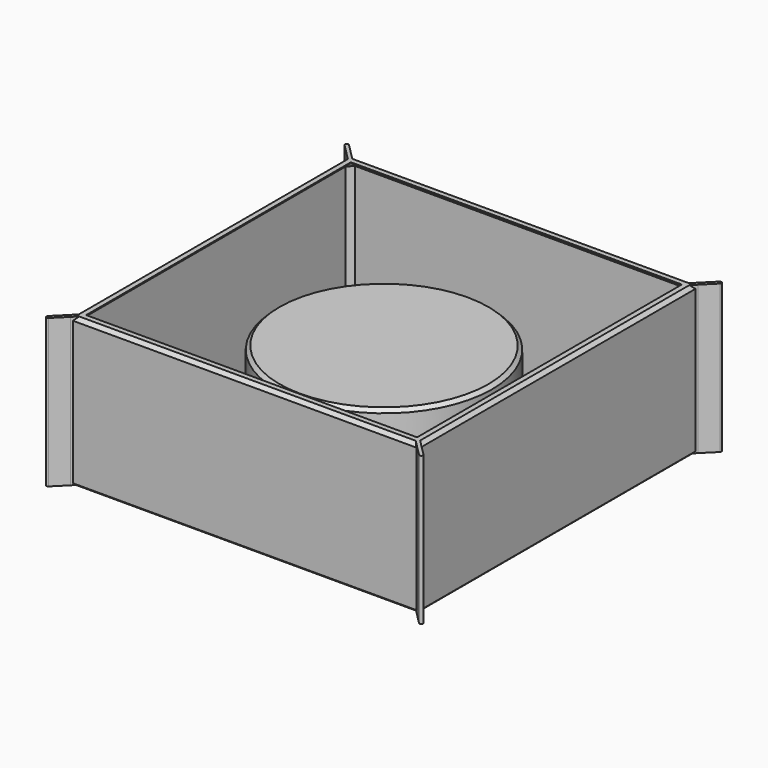
from build123d import *

# Parameters (mm, degrees)
F0_W             = 80
F0_H             = 80
F1_DEPTH         = 34
F2_T             = -0.8
F3_R             = 25
F4_DEPTH         = 24
F4_TAPER         = 0.5
F5_T1_DEPTH      = 78.4
F5_T3_DEPTH      = 78.4
F6_W             = 80
F6_H             = 80
F6_W_2           = 76
F6_H_2           = 76
F7_DEPTH         = 0.05
F8_SIZE          = 1.19999
F11_DEPTH        = 34.05
F11_COPIES_COUNT = 4
F14_SIZE         = 3
F16_SIZE         = 0.4
F17_SIZE         = 0.8


# Not quite as in the source:
# - a fillet or chamfer that OpenCascade refuses, or shapes differently, is made with other operations: its cross-section is extruded or revolved along the edge and cut away or added
# - a fillet or chamfer is up to 0.001 mm smaller than in the source, because OpenCascade refuses the exact size
# - a pattern or mirror of a feature is missing from the dataset's text; its kind, count and spacing are read off the source's solid


with BuildPart() as f1:
    # F0 (on Top) → F1 (new body)
    with BuildSketch(Plane.XY):
        Rectangle(F0_W, F0_H)
    extrude(amount=F1_DEPTH)

    # F2
    f2_openings = [f1.faces().sort_by_distance(p)[0] for p in [
        (0, 0, 34),
    ]]
    offset(amount=F2_T, openings=f2_openings)

    # F3 (on face) → F4 (join)
    with BuildSketch(Plane.XY.offset(0.8)):
        Circle(F3_R)
    extrude(amount=F4_DEPTH, taper=F4_TAPER)

    # F5: chamfer of 1.2 on 5 edges, made by hand

    # F5_s2 → F5_t1 (join)
    with BuildSketch(Plane.XZ.offset(-39.2)):
        Polygon((-39.2, 2), (-38, 0.8), (-39.2, 0.8), align=None)
        Polygon((39.2, 2), (38, 0.8), (39.2, 0.8), align=None)
    extrude(amount=F5_T1_DEPTH)

    # F5_s4 → F5_t3 (join)
    with BuildSketch(Plane.YZ.offset(-39.2)):
        Polygon((-39.2, 2), (-38, 0.8), (-39.2, 0.8), align=None)
        Polygon((39.2, 2), (38, 0.8), (39.2, 0.8), align=None)
    extrude(amount=F5_T3_DEPTH)

    # F5_s5 → F5_t6 (revolve)
    with BuildSketch(Plane.XZ):
        Polygon((26.1895734527, 0.8), (24.989619145, 1.9895281574), (25, 0.8), align=None)
    revolve(axis=Axis((0, 0, 0.8), (0, 0, -1)))

    # F6 (on face) → F7 (join)
    with BuildSketch(Plane.XY.offset(34)):
        Rectangle(F6_W, F6_H)
        Rectangle(F6_W_2, F6_H_2, mode=Mode.SUBTRACT)
    extrude(amount=F7_DEPTH)

    # F8 (size 1.2 in the source; OpenCascade refuses exactly that, so slightly less here)
    f8_edges = [f1.edges().sort_by_distance(p)[0] for p in [
        (0, -39.2, 34),
        (-39.2, 0, 34),
        (-39.2, -39.2, 18),
        (-39.2, 39.2, 18),
        (0, 39.2, 34),
        (39.2, 0, 34),
        (39.2, 39.2, 18),
        (39.2, -39.2, 18),
    ]]
    chamfer(f8_edges, length=F8_SIZE)

    # F9: chamfer of 0.8 on 1 edges, made by hand

    # F9_s1 → F9_t2 (revolve, cut)
    with BuildSketch(Plane.XZ):
        Polygon((24.7975364014, 24.0000304615), (23.990555173, 24.8), (24.790555173, 24.8), align=None)
    revolve(axis=Axis((0, 0, 24.8), (0, 0, -1)), mode=Mode.SUBTRACT)

    # F10 (on face) → F11 (join, through all)
    with BuildSketch(Plane(origin=(0, 0, 0), x_dir=(1, 0, 0), z_dir=(0, 0, -1))):
        with BuildLine():
            Line((-39.1612012219, 39.7268866468), (-39.7171572875, 40.2828427125))
            ThreePointArc((-39.7171572875, 40.2828427125), (-39.7171572875, 39.7171572875), (-40.2828427125, 39.7171572875))
            Line((-40.2828427125, 39.7171572875), (-39.7268866468, 39.1612012219))
            Line((-39.7268866468, 39.1612012219), (-39.1612012219, 39.7268866468))
        make_face()
        with BuildLine():
            ThreePointArc((-40.2828427125, 39.7171572875), (-39.7171572875, 39.7171572875), (-39.7171572875, 40.2828427125))
            Line((-39.7171572875, 40.2828427125), (-42.5455844123, 43.1112698372))
            ThreePointArc((-42.5455844123, 43.1112698372), (-43.1112698372, 43.1112698372), (-43.1112698372, 42.5455844123))
            Line((-43.1112698372, 42.5455844123), (-40.2828427125, 39.7171572875))
        make_face()
    f11 = extrude(amount=-F11_DEPTH)

    # F11_copies: F11 ×4 about axis
    f11_copies_axis = Axis((0, 0, 0), (0, 0, 1))
    for i in range(1, F11_COPIES_COUNT):
        add(f11.rotate(f11_copies_axis, i * 360 / F11_COPIES_COUNT))

    # F12 (on Front) → F13 (revolve, cut)
    with BuildSketch(Plane.XZ):
        Polygon((-23.9975059387, 24.0000304615), (-24.2264749318, -2.2372173829), (0, -2.2372173829), (0, 24.0000304615), align=None)
    revolve(axis=Axis((0, 0, 10.8814065393), (0, 0, 1)), mode=Mode.SUBTRACT)

    # F14
    f14_edges = [f1.edges().sort_by_distance(p)[0] for p in [
        (23.997506, 0, 24.00003),
    ]]
    chamfer(f14_edges, length=F14_SIZE)

    # F15: chamfer of 1.2 on 1 edges, made by hand

    # F15_s1 → F15_t2 (revolve, cut)
    with BuildSketch(Plane.XZ):
        Polygon((-24.1964791889, 1.1999543077), (-25.4069510315, 0), (-24.2069510315, 0), align=None)
    revolve(axis=Axis((0, 0, 0), (0, 0, -1)), mode=Mode.SUBTRACT)

    # F16
    f16_edges = [f1.edges().sort_by_distance(p)[0] for p in [
        (0, -40, 0),
        (-40, 0, 0),
        (40, 0, 0),
        (0, 40, 0),
    ]]
    chamfer(f16_edges, length=F16_SIZE)

    # F17
    f17_edges = [f1.edges().sort_by_distance(p)[0] for p in [
        (0, -40, 34.05),
        (40, 0, 34.05),
        (0, 40, 34.05),
        (-40, 0, 34.05),
    ]]
    chamfer(f17_edges, length=F17_SIZE)


solid = f1.part
